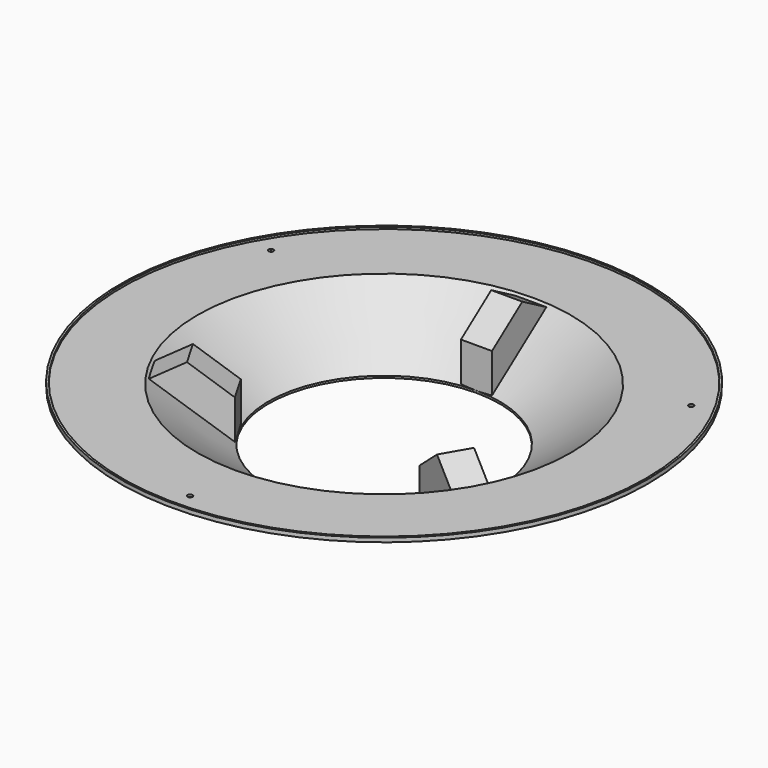
from build123d import *

# Parameters (mm, degrees)
F0_R      = 128.59
F1_DEPTH  = 27.94
F4_T      = 1
F5_D      = 116.84
F5_DEPTH  = 1.001
F7_DEPTH  = 7.625
F8_COUNT  = 3
F8_ANGLE  = 240
F9_R      = 1.25
F10_DEPTH = 34.4029090411


with BuildPart() as f1:
    # F0 (on Top) → F1 (new body)
    with BuildSketch(Plane.XY):
        Circle(F0_R)
    extrude(amount=F1_DEPTH)

    # F2 (on Right) → F3 (revolve, cut)
    with BuildSketch(Plane.YZ):
        Polygon((56.7052650416, 1), (56.7052650416, 0), (128.59, 0), (128.59, 26.94), (91.6200186005, 26.94), align=None)
    revolve(axis=Axis((0, 0, 0), (0, 0, -1)), mode=Mode.SUBTRACT)

    # F4
    f4_openings = [f1.faces().sort_by_distance(p)[0] for p in [
        (0, 0, 27.94),
    ]]
    offset(amount=F4_T, openings=f4_openings, kind=Kind.INTERSECTION)

    # F5 (through all, one way)
    with BuildSketch(Plane.XY):
        with Locations((0, 0)):
            Circle(F5_D / 2)
    extrude(amount=-F5_DEPTH, mode=Mode.SUBTRACT)

    # F6 (on Right) → F7 (join, symmetric)
    with BuildSketch(Plane.YZ):
        Polygon((56.7052650416, 20.6052829476), (56.7052650416, 1), (90.2452650416, 25.9186235421), (75.2752650416, 34.4019090411), align=None)
    extrude(amount=F7_DEPTH, both=True)

    # F8: F1 ×3 about axis
    f8_axis = Axis((0, 0, 0.4971682023), (0, 0, -1))


with BuildPart() as f1_1:
    add(f1.part)
    for i in range(1, F8_COUNT):
        add(f1.part.rotate(f8_axis, i * F8_ANGLE / (F8_COUNT - 1)))

    # F9 (on Top) → F10 (cut, through all)
    with BuildSketch(Plane.XY):
        with Locations((-103.1263050827, 59.54)):
            Circle(F9_R)
        with Locations((0, -119.08)):
            Circle(F9_R)
        with Locations((103.1263050827, 59.54)):
            Circle(F9_R)
    extrude(amount=F10_DEPTH, mode=Mode.SUBTRACT)


solid = f1_1.part
